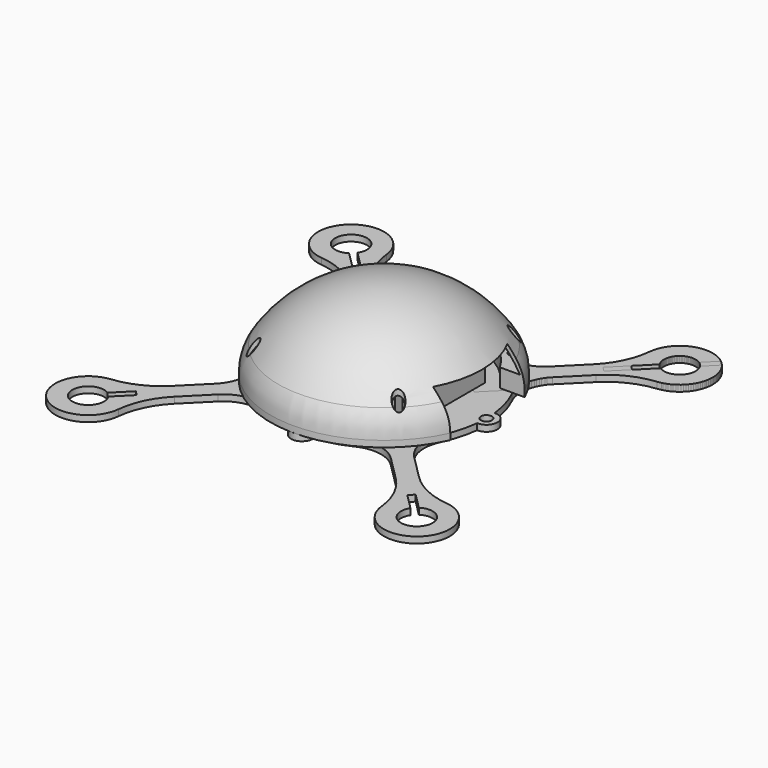
from build123d import *

# Parameters (mm, degrees)
F0_R      = 4.33
F0_R_2    = 1.5
F1_DEPTH  = 1.7
F3_DEPTH  = 12.5
F6_DEPTH  = 12.5
F8_DEPTH  = 12.5
F9_W      = 30.48
F9_H      = 2.54
F10_DEPTH = 8.5
F12_DEPTH = 0.89
F13_R     = 31
F13_R_2   = 1.5
F13_R_3   = 25
F14_DEPTH = 5
F17_R     = 1.5
F18_DEPTH = 25
F20_W     = 25.4
F20_H     = 11.3
F21_DEPTH = 300
F22_W     = 35
F22_H     = 25.4
F23_DEPTH = 11.3


# Not quite as in the source:
# - a fillet or chamfer that OpenCascade refuses, or shapes differently, is made with other operations: its cross-section is extruded or revolved along the edge and cut away or added


with BuildPart() as f1:
    # F0 (on Top) → F1 (new body)
    with BuildSketch(Plane.XY):
        with BuildLine():
            ThreePointArc((-27.1424590693, 23.6069251634), (-24.3536377943, 18.2039662193), (-25.2099671756, 12.1843159432))
            ThreePointArc((-25.2099671756, 12.1843159432), (-26.9195748529, 7.7030182227), (-27.8392857143, 2.99569206))
            ThreePointArc((-27.8392857143, 2.99569206), (-31, 0), (-27.8392857143, -2.99569206))
            ThreePointArc((-27.8392857143, -2.99569206), (-26.9195748529, -7.7030182227), (-25.2099671756, -12.1843159432))
            ThreePointArc((-25.2099671756, -12.1843159432), (-24.3536377943, -18.2039662193), (-27.1424590693, -23.6069251634))
            Line((-27.1424590693, -23.6069251634), (-33.7316985254, -30.1961646194))
            ThreePointArc((-33.7316985254, -30.1961646194), (-39.2820074249, -34.1144972494), (-45.8237972224, -35.9486852782))
            ThreePointArc((-45.8237972224, -35.9486852782), (-51.265241636, -51.265241636), (-35.9486852782, -45.8237972224))
            ThreePointArc((-35.9486852782, -45.8237972224), (-34.1144972494, -39.2820074249), (-30.1961646194, -33.7316985254))
            Line((-30.1961646194, -33.7316985254), (-23.6069251634, -27.1424590693))
            ThreePointArc((-23.6069251634, -27.1424590693), (-18.2039662193, -24.3536377943), (-12.1843159432, -25.2099671756))
            ThreePointArc((-12.1843159432, -25.2099671756), (-7.7030182227, -26.9195748529), (-2.99569206, -27.8392857143))
            ThreePointArc((-2.99569206, -27.8392857143), (-2.2483848126, -27.9095819699), (-1.4994617976, -27.9598214286))
            ThreePointArc((-1.4994617976, -27.9598214286), (0, -26.5), (1.4994617976, -27.9598214286))
            ThreePointArc((1.4994617976, -27.9598214286), (2.2483848126, -27.9095819699), (2.99569206, -27.8392857143))
            ThreePointArc((2.99569206, -27.8392857143), (7.7030182227, -26.9195748529), (12.1843159432, -25.2099671756))
            ThreePointArc((12.1843159432, -25.2099671756), (18.2039662193, -24.3536377943), (23.6069251634, -27.1424590693))
            Line((23.6069251634, -27.1424590693), (30.1961646194, -33.7316985254))
            ThreePointArc((30.1961646194, -33.7316985254), (34.1144972494, -39.2820074249), (35.9486852782, -45.8237972224))
            ThreePointArc((35.9486852782, -45.8237972224), (51.265241636, -51.265241636), (45.8237972224, -35.9486852782))
            ThreePointArc((45.8237972224, -35.9486852782), (39.2820074249, -34.1144972494), (33.7316985254, -30.1961646194))
            Line((33.7316985254, -30.1961646194), (27.1424590693, -23.6069251634))
            ThreePointArc((27.1424590693, -23.6069251634), (24.3536377943, -18.2039662193), (25.2099671756, -12.1843159432))
            ThreePointArc((25.2099671756, -12.1843159432), (26.9195748529, -7.7030182227), (27.8392857143, -2.99569206))
            ThreePointArc((27.8392857143, -2.99569206), (31, 0), (27.8392857143, 2.99569206))
            ThreePointArc((27.8392857143, 2.99569206), (26.9195748529, 7.7030182227), (25.2099671756, 12.1843159432))
            ThreePointArc((25.2099671756, 12.1843159432), (24.3536377943, 18.2039662193), (27.1424590693, 23.6069251634))
            Line((27.1424590693, 23.6069251634), (33.7316985254, 30.1961646194))
            ThreePointArc((33.7316985254, 30.1961646194), (39.2820074249, 34.1144972494), (45.8237972224, 35.9486852782))
            ThreePointArc((45.8237972224, 35.9486852782), (51.265241636, 51.265241636), (35.9486852782, 45.8237972224))
            ThreePointArc((35.9486852782, 45.8237972224), (34.1144972494, 39.2820074249), (30.1961646194, 33.7316985254))
            Line((30.1961646194, 33.7316985254), (23.6069251634, 27.1424590693))
            ThreePointArc((23.6069251634, 27.1424590693), (18.2039662193, 24.3536377943), (12.1843159432, 25.2099671756))
            ThreePointArc((12.1843159432, 25.2099671756), (7.7030182227, 26.9195748529), (2.99569206, 27.8392857143))
            ThreePointArc((2.99569206, 27.8392857143), (0, 31), (-2.99569206, 27.8392857143))
            ThreePointArc((-2.99569206, 27.8392857143), (-7.7030182227, 26.9195748529), (-12.1843159432, 25.2099671756))
            ThreePointArc((-12.1843159432, 25.2099671756), (-18.2039662193, 24.3536377943), (-23.6069251634, 27.1424590693))
            Line((-23.6069251634, 27.1424590693), (-30.1961646194, 33.7316985254))
            ThreePointArc((-30.1961646194, 33.7316985254), (-34.1144972494, 39.2820074249), (-35.9486852782, 45.8237972224))
            ThreePointArc((-35.9486852782, 45.8237972224), (-51.265241636, 51.265241636), (-45.8237972224, 35.9486852782))
            ThreePointArc((-45.8237972224, 35.9486852782), (-39.2820074249, 34.1144972494), (-33.7316985254, 30.1961646194))
            Line((-33.7316985254, 30.1961646194), (-27.1424590693, 23.6069251634))
        make_face()
        with Locations((-44.9012806053, -44.9012806053)):
            Circle(F0_R, mode=Mode.SUBTRACT)
        with Locations((-19.7989898732, -19.7989898732)):
            Circle(F0_R_2, mode=Mode.SUBTRACT)
        with Locations((44.9012806053, -44.9012806053)):
            Circle(F0_R, mode=Mode.SUBTRACT)
        with Locations((19.7989898732, -19.7989898732)):
            Circle(F0_R_2, mode=Mode.SUBTRACT)
        with Locations((-28, 0)):
            Circle(F0_R_2, mode=Mode.SUBTRACT)
        with Locations((-19.7989898732, 19.7989898732)):
            Circle(F0_R_2, mode=Mode.SUBTRACT)
        with Locations((-44.9012806053, 44.9012806053)):
            Circle(F0_R, mode=Mode.SUBTRACT)
        with Locations((19.7989898732, 19.7989898732)):
            Circle(F0_R_2, mode=Mode.SUBTRACT)
        with Locations((28, 0)):
            Circle(F0_R_2, mode=Mode.SUBTRACT)
        with Locations((0, 28)):
            Circle(F0_R_2, mode=Mode.SUBTRACT)
        with Locations((44.9012806053, 44.9012806053)):
            Circle(F0_R, mode=Mode.SUBTRACT)
        with BuildLine():
            ThreePointArc((-1.4994617976, -27.9598214286), (-2.2483848126, -27.9095819699), (-2.99569206, -27.8392857143))
            ThreePointArc((-2.99569206, -27.8392857143), (0, -31), (2.99569206, -27.8392857143))
            ThreePointArc((2.99569206, -27.8392857143), (2.2483848126, -27.9095819699), (1.4994617976, -27.9598214286))
            ThreePointArc((1.4994617976, -27.9598214286), (1.4998654434, -27.979908912), (1.5, -28))
            ThreePointArc((1.5, -28), (-0.020091088, -29.4998654434), (-1.4994617976, -27.9598214286))
        make_face()
    extrude(amount=F1_DEPTH)

    # F2 (on Top) → F3 (cut, symmetric)
    with BuildSketch(Plane.XY):
        Polygon((-45.3043314706, -44.0315392645), (-44.0315392645, -45.3043314706), (-36.9604714526, -38.2332636588), (-38.2332636588, -36.9604714526), align=None)
        Polygon((-38.2332636588, 36.9604714526), (-36.9604714526, 38.2332636588), (-44.0315392645, 45.3043314706), (-45.3043314706, 44.0315392645), align=None)
        Polygon((44.0315392645, -45.3043314706), (45.3043314706, -44.0315392645), (38.2332636588, -36.9604714526), (36.9604714526, -38.2332636588), align=None)
        Polygon((44.0315392645, 45.3043314706), (36.9604714526, 38.2332636588), (38.2332636588, 36.9604714526), (45.3043314706, 44.0315392645), align=None)
    extrude(amount=F3_DEPTH, both=True, mode=Mode.SUBTRACT)


with BuildPart() as f4_1:
    # F4: copy of F1
    add(f1.part)

    # F5 (on Top) → F6 (cut, symmetric)
    with BuildSketch(Plane.XY):
        Polygon((7.8347431355, 18.3282077684), (29.0479465711, 39.541411204), (-36.4159992311, 105.0053570062), (-177.8373554684, -36.4159992311), (-36.4159992311, -177.8373554684), (105.0053570062, -36.4159992311), (39.541411204, 29.0479465711), (18.3282077684, 7.8347431355), align=None)
    extrude(amount=F6_DEPTH, both=True, mode=Mode.SUBTRACT)

    # F7 (on Top) → F8 (cut, symmetric)
    with BuildSketch(Plane.XY):
        Polygon((33.9481965648, 32.6754043586), (38.2332636588, 36.9604714526), (36.9604714526, 38.2332636588), (32.6754043586, 33.9481965648), align=None)
        Polygon((41.2699804971, 42.5427727033), (42.5427727033, 41.2699804971), (56.684908327, 55.4121161209), (55.4121161209, 56.684908327), align=None)
    extrude(amount=F8_DEPTH, both=True, mode=Mode.SUBTRACT)


with BuildPart() as f10:
    # F9 (on face) → F10 (new body)
    with BuildSketch(Plane.XY.offset(1.7)):
        with Locations((0, -13.97)):
            Rectangle(F9_W, F9_H)
    extrude(amount=F10_DEPTH)


with BuildPart() as f10b:
    # F9 (on face) → F10, piece 2 (new body)
    with BuildSketch(Plane.XY.offset(1.7)):
        with Locations((0, 13.97)):
            Rectangle(F9_W, F9_H)
    extrude(amount=F10_DEPTH)


with BuildPart() as f12:
    # F11 (on Right) → F12 (new body, symmetric)
    with BuildSketch(Plane.YZ):
        with BuildLine():
            Line((-6, -3.56), (0, -3.56))
            Line((0, -3.56), (0, 8.16))
            Line((0, 8.16), (8.66, 8.16))
            Line((8.66, 8.16), (8.66, -1.78))
            Line((8.66, -1.78), (11.66, -1.78))
            Line((11.66, -1.78), (11.66, 14.7249563756))
            ThreePointArc((11.66, 14.7249563756), (3.5, 19.97), (-4.66, 14.7249563756))
            ThreePointArc((-4.66, 14.7249563756), (-7.182775387, 6.7971465186), (-11.98, 0))
            Line((-11.98, 0), (-11.98, -1.78))
            Line((-11.98, -1.78), (-6, -1.78))
            Line((-6, -1.78), (-6, -3.56))
        make_face()
    extrude(amount=F12_DEPTH, both=True)


with BuildPart() as f14:
    # F13 (on face) → F14 (new body)
    with BuildSketch(Plane.XY.offset(1.7)):
        Circle(F13_R)
        with Locations((-19.7989898732, -19.7989898732)):
            Circle(F13_R_2, mode=Mode.SUBTRACT)
        with Locations((19.7989898732, -19.7989898732)):
            Circle(F13_R_2, mode=Mode.SUBTRACT)
        with Locations((-19.7989898732, 19.7989898732)):
            Circle(F13_R_2, mode=Mode.SUBTRACT)
        Circle(F13_R_3, mode=Mode.SUBTRACT)
        with Locations((19.7989898732, 19.7989898732)):
            Circle(F13_R_2, mode=Mode.SUBTRACT)
    extrude(amount=F14_DEPTH)

    # F15 (on Front) → F16 (revolve)
    with BuildSketch(Plane.XZ):
        with BuildLine():
            Line((29.8663690461, 6.7), (31, 6.7))
            ThreePointArc((31, 6.7), (18.1151498983, 20.3992326552), (0, 25.4519231907))
            Line((0, 25.4519231907), (0, 24.4519231907))
            ThreePointArc((0, 24.4519231907), (17.3718938013, 19.6789193716), (29.8663690461, 6.7))
        make_face()
    revolve(axis=Axis((0, 0, 16.0759615954), (0, 0, -1)))

    # F17 (on face) → F18 (cut)
    with BuildSketch(Plane(origin=(0, 0, 1.7), x_dir=(1, 0, 0), z_dir=(0, 0, -1))):
        with Locations((19.7989898732, 19.7989898732)):
            Circle(F17_R)
        with Locations((-19.7989898732, 19.7989898732)):
            Circle(F17_R)
        with Locations((19.7989898732, -19.7989898732)):
            Circle(F17_R)
        with Locations((-19.7989898732, -19.7989898732)):
            Circle(F17_R)
    extrude(amount=-F18_DEPTH, mode=Mode.SUBTRACT)

    # F19: fillet of radius 12 on 1 edges, made by hand

    # F19_s1 → F19_t2 (revolve, cut)
    with BuildSketch(Plane.XZ):
        with BuildLine():
            ThreePointArc((31, 3.4134045875), (30.4663970309, 6.9520115353), (28.9130434783, 10.1759166207))
            ThreePointArc((28.9130434783, 10.1759166207), (30.0068941044, 8.468202113), (31, 6.7))
            Line((31, 6.7), (31, 3.4134045875))
        make_face()
    revolve(axis=Axis((0, 0, 6.7), (0, 0, 1)), mode=Mode.SUBTRACT)

    # F20 (on Right) → F21 (cut)
    with BuildSketch(Plane.YZ):
        with Locations((0, 7.35)):
            Rectangle(F20_W, F20_H)
    extrude(amount=F21_DEPTH, mode=Mode.SUBTRACT)


with BuildPart() as f23:
    # F22 (on Top) → F23 (new body)
    with BuildSketch(Plane.XY):
        Rectangle(F22_W, F22_H)
    extrude(amount=F23_DEPTH)


solid = Compound([f1.part, f4_1.part, f10.part, f10b.part, f12.part, f14.part, f23.part])
